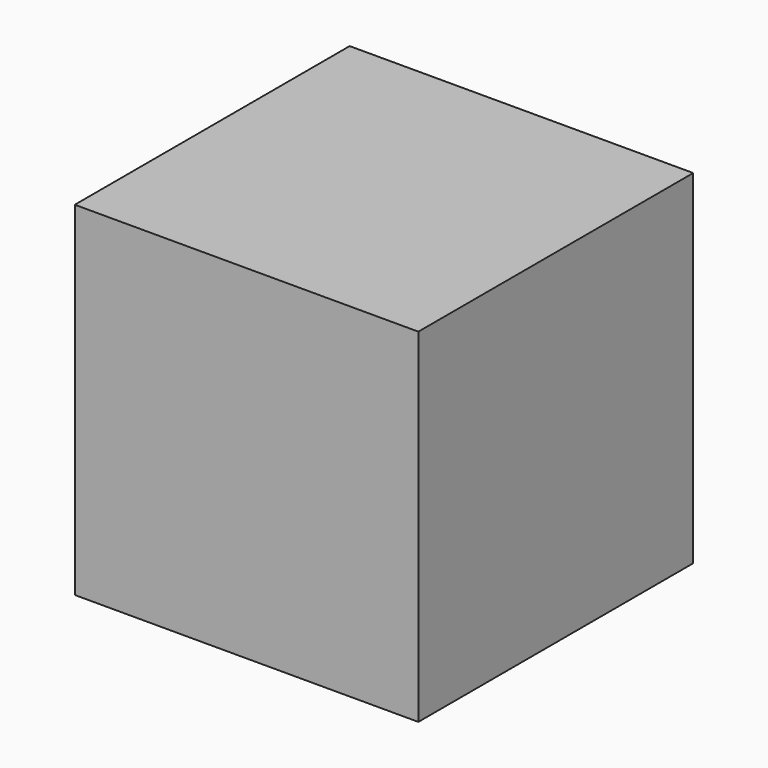
from build123d import *

# Parameters (mm, degrees)
F0_W          = 100
F0_H          = 200
F1_DEPTH      = 1
F1_DEPTH_BACK = 1
F2_W          = 1000
F2_H          = 1000
F3_DEPTH      = 500
F3_DEPTH_BACK = 500


# Not quite as in the source:
# - a feature names something its author has since deleted; it is built from what else it names


with BuildPart() as f1:
    # F0 (on Top) → F1 (new body, two sides)
    with BuildSketch(Plane.XY) as f1_sk:
        Rectangle(F0_W, F0_H)
    extrude(amount=F1_DEPTH)
    extrude(f1_sk.sketch, amount=-F1_DEPTH_BACK)


with BuildPart() as f3:
    # F2 (on Top) → F3 (new body, two sides)
    with BuildSketch(Plane.XY) as f3_sk:
        Rectangle(F2_W, F2_H)
    extrude(amount=F3_DEPTH)
    extrude(f3_sk.sketch, amount=-F3_DEPTH_BACK)

    # F4: cut F1
    add(f1.part, mode=Mode.SUBTRACT)


solid = Compound([f1.part, f3.part])
